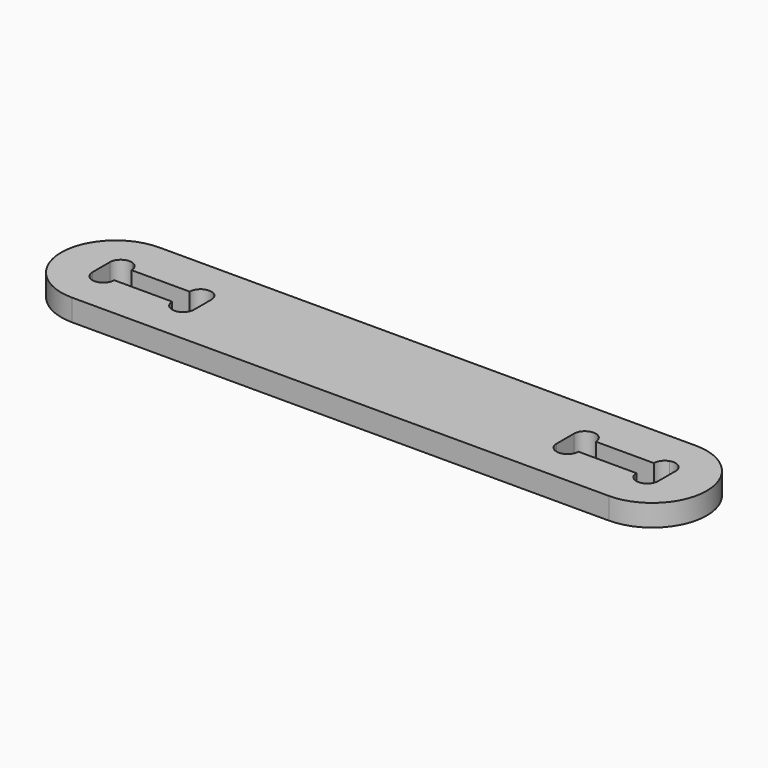
from build123d import *

# Parameters (mm, degrees)
F2_DEPTH = 19.05


# Not quite as in the source:
# - a variable given as a bare number and used for a length is read in inches; the dataset says mm whatever the document's units were


with BuildPart() as f2:
    # F1 (on Top) → F2 (new body)
    with BuildSketch(Plane.XY):
        with BuildLine():
            Line((234.95, 47.625), (-234.95, 47.625))
            Line((-234.95, 47.625), (-234.95, 18.5052561211))
            ThreePointArc((-234.95, 18.5052561211), (-230.3478700667, 15.024261314), (-228.6, 9.525))
            Line((-228.6, 9.525), (-177.8, 9.525))
            ThreePointArc((-177.8, 9.525), (-168.275, 19.05), (-158.75, 9.525))
            Line((-158.75, 9.525), (-158.75, -9.525))
            ThreePointArc((-158.75, -9.525), (-168.275, -19.05), (-177.8, -9.525))
            Line((-177.8, -9.525), (-228.6, -9.525))
            ThreePointArc((-228.6, -9.525), (-230.3478700667, -15.024261314), (-234.95, -18.5052561211))
            Line((-234.95, -18.5052561211), (-234.95, -47.625))
            Line((-234.95, -47.625), (234.95, -47.625))
            Line((234.95, -47.625), (234.95, -18.5052561211))
            ThreePointArc((234.95, -18.5052561211), (230.3478700667, -15.024261314), (228.6, -9.525))
            Line((228.6, -9.525), (177.8, -9.525))
            ThreePointArc((177.8, -9.525), (168.275, -19.05), (158.75, -9.525))
            Line((158.75, -9.525), (158.75, 9.525))
            ThreePointArc((158.75, 9.525), (168.275, 19.05), (177.8, 9.525))
            Line((177.8, 9.525), (228.6, 9.525))
            ThreePointArc((228.6, 9.525), (230.3478700667, 15.024261314), (234.95, 18.5052561211))
            Line((234.95, 18.5052561211), (234.95, 47.625))
        make_face()
        with BuildLine():
            Line((-234.95, 18.5052561211), (-234.95, 47.625))
            ThreePointArc((-234.95, 47.625), (-282.575, 0), (-234.95, -47.625))
            Line((-234.95, -47.625), (-234.95, -18.5052561211))
            ThreePointArc((-234.95, -18.5052561211), (-243.624261314, -17.3021299333), (-247.65, -9.525))
            Line((-247.65, -9.525), (-247.65, 9.525))
            ThreePointArc((-247.65, 9.525), (-243.624261314, 17.3021299333), (-234.95, 18.5052561211))
        make_face()
        with BuildLine():
            ThreePointArc((234.95, -47.625), (282.575, 0), (234.95, 47.625))
            Line((234.95, 47.625), (234.95, 18.5052561211))
            ThreePointArc((234.95, 18.5052561211), (243.624261314, 17.3021299333), (247.65, 9.525))
            Line((247.65, 9.525), (247.65, -9.525))
            ThreePointArc((247.65, -9.525), (243.624261314, -17.3021299333), (234.95, -18.5052561211))
            Line((234.95, -18.5052561211), (234.95, -47.625))
        make_face()
    extrude(amount=F2_DEPTH)


solid = f2.part
